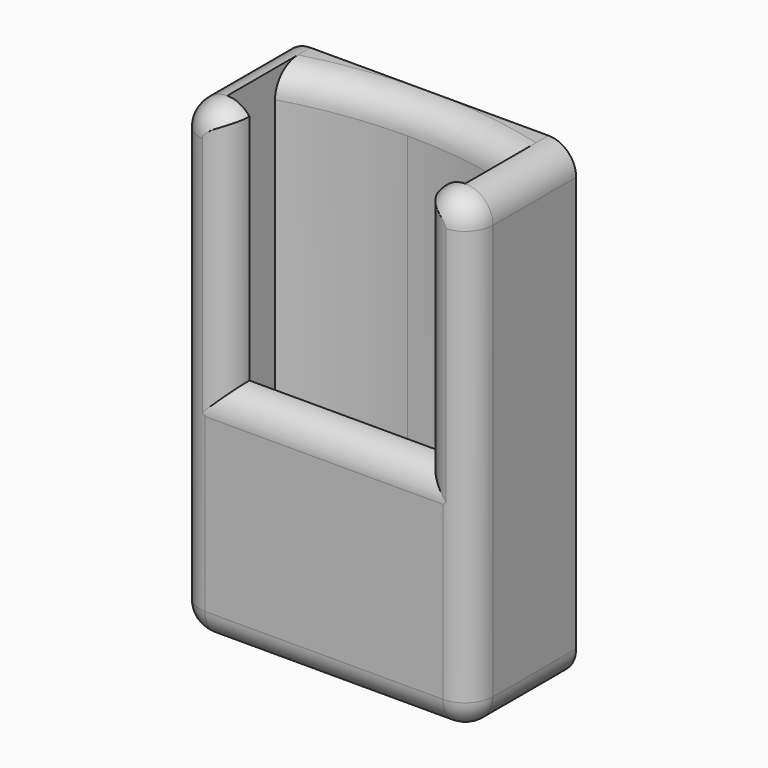
from build123d import *

# Parameters (mm, degrees)
F0_W         = 53
F0_H         = 23.8
F0_W_2       = 43
F0_H_2       = 13.8
F1_DEPTH     = 80
F2_DEPTH     = 5
F3_W         = 35
F3_H         = 44
F4_DEPTH     = 25
F5_T1_DEPTH  = 78
F5_T3_DEPTH  = 110
F5_T5_DEPTH  = 35
F5_T7_DEPTH  = 56.5
F5_T13_DEPTH = 69
F5_T17_DEPTH = 47.5
F5_T24_DEPTH = 47.5
F5_T28_DEPTH = 69
F6_T1_DEPTH  = 31.3
F6_S5_W      = 5
F6_S5_H      = 5
F6_T6_DEPTH  = 5
F6_S11_W     = 5
F6_S11_H     = 5
F6_T12_DEPTH = 5
F7_R         = 4.99999
F9_DEPTH     = 80
F10_T4_ANGLE = 50.0121835392


# Not quite as in the source:
# - a fillet or chamfer that OpenCascade refuses, or shapes differently, is made with other operations: its cross-section is extruded or revolved along the edge and cut away or added
# - a fillet or chamfer is up to 0.001 mm smaller than in the source, because OpenCascade refuses the exact size


with BuildPart() as f1:
    # F0 (on Top) → F1 (new body)
    with BuildSketch(Plane.XY):
        with Locations((-2.25, 0.0045082584)):
            Rectangle(F0_W, F0_H)
        with Locations((-2.25, 0.0045082584)):
            Rectangle(F0_W_2, F0_H_2, mode=Mode.SUBTRACT)
    extrude(amount=F1_DEPTH)

    # F0 (on Top) → F2 (join)
    with BuildSketch(Plane.XY):
        with Locations((-2.25, 0.0045082584)):
            Rectangle(F0_W, F0_H)
        with Locations((-2.25, 0.0045082584)):
            Rectangle(F0_W_2, F0_H_2, mode=Mode.SUBTRACT)
        with Locations((-2.25, 0.0045082584)):
            Rectangle(F0_W_2, F0_H_2)
    extrude(amount=-F2_DEPTH)

    # F3 (on face) → F4 (cut)
    with BuildSketch(Plane(origin=(0, -6.8954917416, 0), x_dir=(-1, 0, 0), z_dir=(0, 1, 0))):
        with Locations((2.25, 58)):
            Rectangle(F3_W, F3_H)
    extrude(amount=-F4_DEPTH, mode=Mode.SUBTRACT)

    # F5: fillet of radius 5 on 6 edges, made by hand

    # F5_s2 → F5_t1 (cut)
    with BuildSketch(Plane.YZ.offset(-41.25)):
        with BuildLine():
            ThreePointArc((-11.8954917416, 0), (-10.4310256475, -3.5355339059), (-6.8954917416, -5))
            Line((-6.8954917416, -5), (-11.8954917416, -5))
            Line((-11.8954917416, -5), (-11.8954917416, 0))
        make_face()
    extrude(amount=F5_T1_DEPTH, mode=Mode.SUBTRACT)

    # F5_s4 → F5_t3 (cut)
    with BuildSketch(Plane.XY.offset(-17.5)):
        with BuildLine():
            ThreePointArc((-23.75, -11.8954917416), (-27.2855339059, -10.4310256475), (-28.75, -6.8954917416))
            Line((-28.75, -6.8954917416), (-28.75, -11.8954917416))
            Line((-28.75, -11.8954917416), (-23.75, -11.8954917416))
        make_face()
        with BuildLine():
            ThreePointArc((24.25, -6.8954917416), (22.7855339059, -10.4310256475), (19.25, -11.8954917416))
            Line((19.25, -11.8954917416), (24.25, -11.8954917416))
            Line((24.25, -11.8954917416), (24.25, -6.8954917416))
        make_face()
    extrude(amount=F5_T3_DEPTH, mode=Mode.SUBTRACT)

    # F5_s6 → F5_t5 (cut)
    with BuildSketch(Plane.YZ.offset(-19.75)):
        with BuildLine():
            ThreePointArc((-11.8954917416, 31), (-10.4310256475, 34.5355339059), (-6.8954917416, 36))
            Line((-6.8954917416, 36), (-11.8954917416, 36))
            Line((-11.8954917416, 36), (-11.8954917416, 31))
        make_face()
    extrude(amount=F5_T5_DEPTH, mode=Mode.SUBTRACT)

    # F5_s8 → F5_t7 (cut)
    with BuildSketch(Plane.XY.offset(36)):
        with BuildLine():
            ThreePointArc((-24.75, -11.8954917416), (-21.2144660941, -10.4310256475), (-19.75, -6.8954917416))
            Line((-19.75, -6.8954917416), (-19.75, -11.8954917416))
            Line((-19.75, -11.8954917416), (-24.75, -11.8954917416))
        make_face()
        with BuildLine():
            ThreePointArc((20.25, -11.8954917416), (16.7144660941, -10.4310256475), (15.25, -6.8954917416))
            Line((15.25, -6.8954917416), (15.25, -11.8954917416))
            Line((15.25, -11.8954917416), (20.25, -11.8954917416))
        make_face()
    extrude(amount=F5_T7_DEPTH, mode=Mode.SUBTRACT)


with BuildPart() as f5_tool11:
    # F5_s12 → F5_t13 (new body)
    with BuildSketch(Plane.XY.offset(92.5)):
        with BuildLine():
            ThreePointArc((20.25, -11.8954917416), (16.7144660941, -10.4310256475), (15.25, -6.8954917416))
            Line((15.25, -6.8954917416), (15.25, -11.8954917416))
            Line((15.25, -11.8954917416), (20.25, -11.8954917416))
        make_face()
    extrude(amount=-F5_T13_DEPTH)

    split(bisect_by=Plane.XY.offset(36), keep=Keep.BOTTOM)


with BuildPart() as f5_tool15:
    # F5_s16 → F5_t17 (new body)
    with BuildSketch(Plane.YZ.offset(27.75)):
        with BuildLine():
            ThreePointArc((-11.8954917416, 31), (-10.4310256475, 34.5355339059), (-6.8954917416, 36))
            Line((-6.8954917416, 36), (-11.8954917416, 36))
            Line((-11.8954917416, 36), (-11.8954917416, 31))
        make_face()
    extrude(amount=-F5_T17_DEPTH)

    split(bisect_by=Plane.YZ.offset(15.25), keep=Keep.TOP)


with BuildPart() as f5_tool11_1:
    add(f5_tool11.part)

    # F5_t19: intersect F5_tool15
    add(f5_tool15.part, mode=Mode.INTERSECT)


with BuildPart() as f1_1:
    add(f1.part)

    # F5_t9: cut F5_tool11
    add(f5_tool11_1.part, mode=Mode.SUBTRACT)


with BuildPart() as f5_tool22:
    # F5_s23 → F5_t24 (new body)
    with BuildSketch(Plane.YZ.offset(15.25)):
        with BuildLine():
            ThreePointArc((-11.8954917416, 31), (-10.4310256475, 34.5355339059), (-6.8954917416, 36))
            Line((-6.8954917416, 36), (-11.8954917416, 36))
            Line((-11.8954917416, 36), (-11.8954917416, 31))
        make_face()
    extrude(amount=-F5_T24_DEPTH)

    split(bisect_by=Plane.YZ.offset(-19.75), keep=Keep.BOTTOM)


with BuildPart() as f5_tool26:
    # F5_s27 → F5_t28 (new body)
    with BuildSketch(Plane.XY.offset(23.5)):
        with BuildLine():
            ThreePointArc((-24.75, -11.8954917416), (-21.2144660941, -10.4310256475), (-19.75, -6.8954917416))
            Line((-19.75, -6.8954917416), (-19.75, -11.8954917416))
            Line((-19.75, -11.8954917416), (-24.75, -11.8954917416))
        make_face()
    extrude(amount=F5_T28_DEPTH)

    split(bisect_by=Plane.XY.offset(36), keep=Keep.BOTTOM)


with BuildPart() as f5_tool22_1:
    add(f5_tool22.part)

    # F5_t30: intersect F5_tool26
    add(f5_tool26.part, mode=Mode.INTERSECT)


with BuildPart() as f1_2:
    add(f1_1.part)

    # F5_t20: cut F5_tool22
    add(f5_tool22_1.part, mode=Mode.SUBTRACT)

    # F6: fillet of radius 5 on 2 edges, made by hand

    # F6_s2 → F6_t1 (cut)
    with BuildSketch(Plane.XZ.offset(-24.4045082584)):
        with BuildLine():
            ThreePointArc((24.25, 0), (22.7855339059, -3.5355339059), (19.25, -5))
            Line((19.25, -5), (24.25, -5))
            Line((24.25, -5), (24.25, 0))
        make_face()
        with BuildLine():
            ThreePointArc((-28.75, 0), (-27.2855339059, -3.5355339059), (-23.75, -5))
            Line((-23.75, -5), (-28.75, -5))
            Line((-28.75, -5), (-28.75, 0))
        make_face()
    extrude(amount=F6_T1_DEPTH, mode=Mode.SUBTRACT)


with BuildPart() as f6_tool4:
    # F6_s5 → F6_t6 (new body)
    with BuildSketch(Plane.YZ.offset(-23.75)):
        with Locations((-9.3954917416, -2.5)):
            Rectangle(F6_S5_W, F6_S5_H)
    extrude(amount=-F6_T6_DEPTH)

    # F6_s7 → F6_t8 (revolve, cut)
    with BuildSketch(Plane(origin=(-23.75, -6.8954917416, 0), x_dir=(0, 0.7071067812, 0.7071067812), z_dir=(0, -0.7071067812, 0.7071067812))):
        with BuildLine():
            ThreePointArc((0, -5), (5, 0), (0, 5))
            Line((0, 5), (0, -5))
        make_face()
    revolve(axis=Axis((-23.75, -6.8954917416, 0), (-1, 0, 0)), mode=Mode.SUBTRACT)


with BuildPart() as f1_3:
    add(f1_2.part)

    # F6_t3: cut F6_tool4
    add(f6_tool4.part, mode=Mode.SUBTRACT)


with BuildPart() as f6_tool10:
    # F6_s11 → F6_t12 (new body)
    with BuildSketch(Plane.YZ.offset(19.25)):
        with Locations((-9.3954917416, -2.5)):
            Rectangle(F6_S11_W, F6_S11_H)
    extrude(amount=F6_T12_DEPTH)

    # F6_s13 → F6_t14 (revolve, cut)
    with BuildSketch(Plane(origin=(19.25, -6.8954917416, 0), x_dir=(0, 0.7071067812, 0.7071067812), z_dir=(0, 0.7071067812, -0.7071067812))):
        with BuildLine():
            ThreePointArc((0, -5), (5, 0), (0, 5))
            Line((0, 5), (0, -5))
        make_face()
    revolve(axis=Axis((19.25, -6.8954917416, 0), (1, 0, 0)), mode=Mode.SUBTRACT)


with BuildPart() as f1_4:
    add(f1_3.part)

    # F6_t9: cut F6_tool10
    add(f6_tool10.part, mode=Mode.SUBTRACT)

    # F7 (radius 5 in the source; OpenCascade refuses exactly that, so slightly less here)
    f7_edges = [f1_4.edges().sort_by_distance(p)[0] for p in [
        (22.958099, -10.249594, 80),
        (-28.75, 2.504508, 80),
    ]]
    fillet(f7_edges, radius=F7_R)

    # F8 (on face) → F9 (join)
    with BuildSketch(Plane.XY):
        with BuildLine():
            ThreePointArc((-2.25, 6.9045082584), (8.604146673, 6.1508927486), (19.25, 3.9045082584))
            Line((19.25, 3.9045082584), (19.25, 6.9045082584))
            Line((19.25, 6.9045082584), (-2.25, 6.9045082584))
        make_face()
        with BuildLine():
            ThreePointArc((-23.75, 3.9045082584), (-13.104146673, 6.1508927486), (-2.25, 6.9045082584))
            Line((-2.25, 6.9045082584), (-23.75, 6.9045082584))
            Line((-23.75, 6.9045082584), (-23.75, 3.9045082584))
        make_face()
    extrude(amount=F9_DEPTH)

    # F10: fillet of radius 5 on 1 edges, made by hand


with BuildPart() as f10_tool2:
    # F10_s3 → F10_t4 (revolve)
    with BuildSketch(Plane(origin=(-29.2914715623, -13.6626291921, 0), x_dir=(0, 0, 1), z_dir=(-0.9062628485, -0.4227146193, 0))):
        with BuildLine():
            ThreePointArc((75, 14.5706793202), (78.5355339059, 16.0351454142), (80, 19.5706793202))
            Line((80, 19.5706793202), (80, 14.5706793202))
            Line((80, 14.5706793202), (75, 14.5706793202))
        make_face()
    revolve(axis=Axis((-2.25, -71.6371584083, 80), (0, 0, -1)), revolution_arc=F10_T4_ANGLE)

    split(bisect_by=Plane.YZ.offset(19.25), keep=Keep.BOTTOM)

    split(bisect_by=Plane.YZ.offset(-23.75), keep=Keep.TOP)


with BuildPart() as f1_5:
    add(f1_4.part)

    # F10_t1: cut F10_tool2
    add(f10_tool2.part, mode=Mode.SUBTRACT)


solid = f1_5.part
